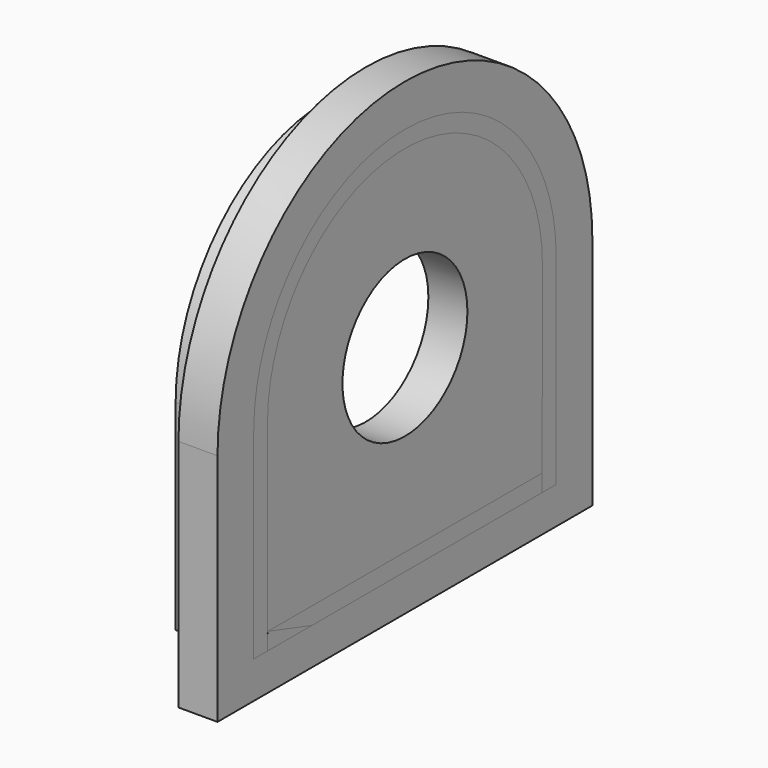
from build123d import *

# Parameters (mm, degrees)
F0_R     = 5
F1_DEPTH = 2.5
F2_DEPTH = 5
F3_DEPTH = 5


# Not quite as in the source:
# - a feature names something its author has since deleted; it is built from what else it names


with BuildPart() as f1:
    # F0 (on Right) → F1 (new body)
    with BuildSketch(Plane.YZ):
        with BuildLine():
            Line((1.875, -4.4410212704), (1.875, 5.5589787296))
            ThreePointArc((1.875, 5.5589787296), (-13.125, 20.5589787296), (-28.125, 5.5589787296))
            Line((-28.125, 5.5589787296), (-28.125, -9.4410212704))
            Line((-28.125, -9.4410212704), (1.875, -9.4410212704))
            Line((1.875, -9.4410212704), (1.875, -4.4410212704))
        make_face()
        with BuildLine():
            ThreePointArc((-0.6214854401, 5.7639283943), (-0.6214854576, 5.7632668705), (-0.6214855101, 5.7626053467))
            Line((-0.6214855101, 5.7626053467), (-0.6214855101, -7.441388098))
            Line((-0.6214855101, -7.441388098), (-1.0466333126, -7.4412858417))
            Line((-1.0466333126, -7.4412858417), (-2.1466328087, -7.4410212704))
            Line((-2.1466328087, -7.4410212704), (-24.1033577683, -7.4357402504))
            Line((-24.1033577683, -7.4357402504), (-25.2253250397, -7.4354703954))
            Line((-25.2253250397, -7.4354703954), (-25.6253250397, -7.4353741876))
            Line((-25.6253250397, -7.4353741876), (-25.6253250397, 5.7652514419))
            ThreePointArc((-25.6253250397, 5.7652514419), (-13.1227437511, 18.2658482116), (-0.6214854401, 5.7639283943))
        make_face(mode=Mode.SUBTRACT)
        with BuildLine():
            ThreePointArc((-8.825371599, -5.9759567979), (-4.9508229486, -3.6968800238), (-2.1328316515, -0.1947030957))
            Line((-2.1328316515, -0.1947030957), (-2.1214855101, 5.7626053467))
            ThreePointArc((-2.1214855101, 5.7626053467), (-13.1220798645, 16.7854966034), (-24.1253250397, 5.7652514419))
            Line((-24.1253250397, 5.7652514419), (-24.1154117036, -0.192059557))
            ThreePointArc((-24.1154117036, -0.192059557), (-21.2994002975, -3.6939309404), (-17.4270857953, -5.9738879181))
            Line((-17.4270857953, -5.9738879181), (-8.825371599, -5.9759567979))
        make_face()
        with Locations((-13.125, 5.5589787296)):
            Circle(F0_R, mode=Mode.SUBTRACT)
        with BuildLine():
            ThreePointArc((-25.2253250397, 2.6268061761), (-25.5250055228, 4.1833243656), (-25.6253249696, 5.7652514419))
            Line((-25.6253250397, 5.7652514419), (-25.6253250397, -7.4353741876))
            Line((-25.6253250397, -7.4353741876), (-25.2253250397, -7.4354703954))
            Line((-25.2253250397, -7.4354703954), (-25.2253250397, -7.0720094287))
            Line((-25.2253250397, -7.0720094287), (-25.2253250397, 2.6268061761))
        make_face()
        with BuildLine():
            Line((-2.1214855101, 5.7626053467), (-1.0214855101, 5.7626053467))
            ThreePointArc((-1.0214855101, 5.7626053467), (-13.1220822273, 17.8658481591), (-25.2253250397, 5.7652514419))
            Line((-25.2253250397, 5.7652514419), (-24.1253250397, 5.7652514419))
            ThreePointArc((-24.1253250397, 5.7652514419), (-13.1220798645, 16.7854966034), (-2.1214855101, 5.7626053467))
        make_face()
        with BuildLine():
            Line((-1.0214855101, 5.7626053467), (-0.6214855101, 5.7626053467))
            ThreePointArc((-0.6214855101, 5.7626053467), (-0.6214854576, 5.7632668705), (-0.6214854401, 5.7639283943))
            ThreePointArc((-0.6214854401, 5.7639283943), (-13.1227437511, 18.2658482116), (-25.6253250397, 5.7652514419))
            Line((-25.6253250397, 5.7652514419), (-25.2253250397, 5.7652514419))
            ThreePointArc((-25.2253250397, 5.7652514419), (-13.1220822273, 17.8658481591), (-1.0214855101, 5.7626053467))
        make_face()
        with BuildLine():
            Line((-25.2253250397, 5.7652514419), (-25.6253250397, 5.7652514419))
            ThreePointArc((-25.6253249696, 5.7652514419), (-25.5250055228, 4.1833243656), (-25.2253250397, 2.6268061761))
            Line((-25.2253250397, 2.6268061761), (-25.2253250397, 5.7652514419))
        make_face()
        with BuildLine():
            Line((-24.1253250397, 5.7652514419), (-25.2253250397, 5.7652514419))
            Line((-25.2253250397, 5.7652514419), (-25.2253250397, 2.6268061761))
            ThreePointArc((-25.2253250397, 2.6268061761), (-24.7560686742, 1.1836292728), (-24.1154117036, -0.192059557))
            Line((-24.1154117036, -0.192059557), (-24.1253250397, 5.7652514419))
        make_face()
        Polygon((-24.1033577683, -7.4357402504), (-2.1466328087, -7.4410212704), (-2.1459405703, -7.0775604702), (-2.1466328087, -7.0775603037), (-20.5701562872, -7.0731290875), (-24.1039625902, -7.0722791382), align=None)
        Polygon((-24.1033577683, -5.9722821446), (-24.1040233922, -7.0357408042), (-24.1039625902, -7.0722791382), (-20.5701562872, -7.0731290875), align=None)
        with BuildLine():
            ThreePointArc((-17.4270857953, -5.9738879181), (-13.12641223, -6.7379910088), (-8.825371599, -5.9759567979))
            Line((-8.825371599, -5.9759567979), (-17.4270857953, -5.9738879181))
        make_face()
        Polygon((-25.2253250397, -7.0720094287), (-25.2253250397, -7.4354703954), (-24.1033577683, -7.4357402504), (-24.1039625902, -7.0722791382), align=None)
        with BuildLine():
            ThreePointArc((-24.1154117036, -0.192059557), (-24.7560686742, 1.1836292728), (-25.2253250397, 2.6268061761))
            Line((-25.2253250397, 2.6268061761), (-25.2253250397, -7.0720094287))
            Line((-25.2253250397, -7.0720094287), (-24.1039625902, -7.0722791382))
            Line((-24.1039625902, -7.0722791382), (-24.1040233922, -7.0357408042))
            Line((-24.1040233922, -7.0357408042), (-24.1154117036, -0.192059557))
        make_face()
        with BuildLine():
            Line((-0.6214855101, -7.441388098), (-0.6214855101, 5.7626053467))
            ThreePointArc((-0.6214855801, 5.7626053467), (-0.7234893636, 4.1701645483), (-1.0275019055, 2.6036879789))
            Line((-1.0275019055, 2.6036879789), (-1.0459410742, -7.0778250415))
            Line((-1.0459410742, -7.0778250415), (-1.0466333126, -7.4412858417))
            Line((-1.0466333126, -7.4412858417), (-0.6214855101, -7.441388098))
        make_face()
        with BuildLine():
            ThreePointArc((-1.0275019055, 2.6036879789), (-0.7234893636, 4.1701645483), (-0.6214855801, 5.7626053467))
            Line((-0.6214855101, 5.7626053467), (-1.0214855101, 5.7626053467))
            Line((-1.0214855101, 5.7626053467), (-1.0275019055, 2.6036879789))
        make_face()
        with BuildLine():
            ThreePointArc((-2.1328316515, -0.1947030957), (-1.495675353, 1.1711193771), (-1.0275019055, 2.6036879789))
            Line((-1.0275019055, 2.6036879789), (-1.0214855101, 5.7626053467))
            Line((-1.0214855101, 5.7626053467), (-2.1214855101, 5.7626053467))
            Line((-2.1214855101, 5.7626053467), (-2.1328316515, -0.1947030957))
        make_face()
        with BuildLine():
            Line((-1.0459410742, -7.0778250415), (-1.0275019055, 2.6036879789))
            ThreePointArc((-1.0275019055, 2.6036879789), (-1.495675353, 1.1711193771), (-2.1328316515, -0.1947030957))
            Line((-2.1328316515, -0.1947030957), (-2.1438455441, -5.977563835))
            Line((-2.1438455441, -5.977563835), (-2.1459405703, -7.0775604702))
            Line((-2.1459405703, -7.0775604702), (-1.0459410742, -7.0778250415))
        make_face()
        with BuildLine():
            Line((-2.1438455441, -5.977563835), (-2.1328316515, -0.1947030957))
            ThreePointArc((-2.1328316515, -0.1947030957), (-4.9508229486, -3.6968800238), (-8.825371599, -5.9759567979))
            Line((-8.825371599, -5.9759567979), (-2.1438455441, -5.977563835))
        make_face()
        Polygon((-2.1466328087, -7.4410212704), (-1.0466333126, -7.4412858417), (-1.0459410742, -7.0778250415), (-2.1459405703, -7.0775604702), align=None)
        with BuildLine():
            ThreePointArc((-17.4270857953, -5.9738879181), (-21.2994002975, -3.6939309404), (-24.1154117036, -0.192059557))
            Line((-24.1154117036, -0.192059557), (-24.1040233922, -7.0357408042))
            Line((-24.1040233922, -7.0357408042), (-24.1033577683, -5.9722821446))
            Line((-24.1033577683, -5.9722821446), (-17.4270857953, -5.9738879181))
        make_face()
        Polygon((-20.5701562872, -7.0731290875), (-17.4270857953, -5.9738879181), (-24.1033577683, -5.9722821446), align=None)
        with BuildLine():
            Line((-2.1438455441, -5.977563835), (-8.825371599, -5.9759567979))
            ThreePointArc((-8.825371599, -5.9759567979), (-13.12641223, -6.7379910088), (-17.4270857953, -5.9738879181))
            Line((-17.4270857953, -5.9738879181), (-20.5701562872, -7.0731290875))
            Line((-20.5701562872, -7.0731290875), (-2.1466328087, -7.0775603037))
            Line((-2.1466328087, -7.0775603037), (-2.1438455441, -5.977563835))
        make_face()
    extrude(amount=-F1_DEPTH)


with BuildPart() as f2:
    # F0 (on Right) → F2 (new body)
    with BuildSketch(Plane.YZ):
        with BuildLine():
            Line((-24.1253250397, 5.7652514419), (-25.2253250397, 5.7652514419))
            Line((-25.2253250397, 5.7652514419), (-25.2253250397, 2.6268061761))
            ThreePointArc((-25.2253250397, 2.6268061761), (-24.7560686742, 1.1836292728), (-24.1154117036, -0.192059557))
            Line((-24.1154117036, -0.192059557), (-24.1253250397, 5.7652514419))
        make_face()
        with BuildLine():
            Line((-2.1214855101, 5.7626053467), (-1.0214855101, 5.7626053467))
            ThreePointArc((-1.0214855101, 5.7626053467), (-13.1220822273, 17.8658481591), (-25.2253250397, 5.7652514419))
            Line((-25.2253250397, 5.7652514419), (-24.1253250397, 5.7652514419))
            ThreePointArc((-24.1253250397, 5.7652514419), (-13.1220798645, 16.7854966034), (-2.1214855101, 5.7626053467))
        make_face()
        with BuildLine():
            ThreePointArc((-2.1328316515, -0.1947030957), (-1.495675353, 1.1711193771), (-1.0275019055, 2.6036879789))
            Line((-1.0275019055, 2.6036879789), (-1.0214855101, 5.7626053467))
            Line((-1.0214855101, 5.7626053467), (-2.1214855101, 5.7626053467))
            Line((-2.1214855101, 5.7626053467), (-2.1328316515, -0.1947030957))
        make_face()
        with BuildLine():
            Line((-1.0459410742, -7.0778250415), (-1.0275019055, 2.6036879789))
            ThreePointArc((-1.0275019055, 2.6036879789), (-1.495675353, 1.1711193771), (-2.1328316515, -0.1947030957))
            Line((-2.1328316515, -0.1947030957), (-2.1438455441, -5.977563835))
            Line((-2.1438455441, -5.977563835), (-2.1459405703, -7.0775604702))
            Line((-2.1459405703, -7.0775604702), (-1.0459410742, -7.0778250415))
        make_face()
        with BuildLine():
            ThreePointArc((-24.1154117036, -0.192059557), (-24.7560686742, 1.1836292728), (-25.2253250397, 2.6268061761))
            Line((-25.2253250397, 2.6268061761), (-25.2253250397, -7.0720094287))
            Line((-25.2253250397, -7.0720094287), (-24.1039625902, -7.0722791382))
            Line((-24.1039625902, -7.0722791382), (-24.1040233922, -7.0357408042))
            Line((-24.1040233922, -7.0357408042), (-24.1154117036, -0.192059557))
        make_face()
    extrude(amount=-F2_DEPTH)


with BuildPart() as f2b:
    # F0 (on Right) → F2, piece 2 (new body)
    with BuildSketch(Plane.YZ):
        with BuildLine():
            ThreePointArc((-17.4270857953, -5.9738879181), (-13.12641223, -6.7379910088), (-8.825371599, -5.9759567979))
            Line((-8.825371599, -5.9759567979), (-17.4270857953, -5.9738879181))
        make_face()
        Polygon((-20.5701562872, -7.0731290875), (-17.4270857953, -5.9738879181), (-24.1033577683, -5.9722821446), align=None)
        with BuildLine():
            Line((-2.1438455441, -5.977563835), (-8.825371599, -5.9759567979))
            ThreePointArc((-8.825371599, -5.9759567979), (-13.12641223, -6.7379910088), (-17.4270857953, -5.9738879181))
            Line((-17.4270857953, -5.9738879181), (-20.5701562872, -7.0731290875))
            Line((-20.5701562872, -7.0731290875), (-2.1466328087, -7.0775603037))
            Line((-2.1466328087, -7.0775603037), (-2.1438455441, -5.977563835))
        make_face()
    extrude(amount=-F2_DEPTH)


with BuildPart() as f3:
    # F0 (on Right) → F3 (new body)
    with BuildSketch(Plane.YZ):
        Polygon((-24.1033577683, -5.9722821446), (-24.1040233922, -7.0357408042), (-24.1039625902, -7.0722791382), (-20.5701562872, -7.0731290875), align=None)
    extrude(amount=-F3_DEPTH)


solid = Compound([f1.part, f2.part, f2b.part, f3.part])
